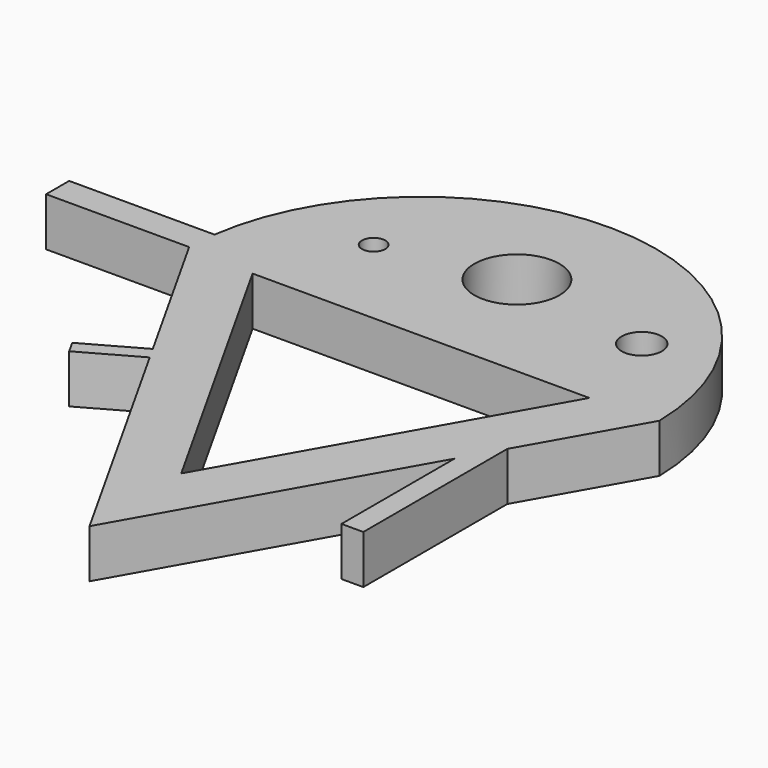
from build123d import *

# Parameters (mm, degrees)
F0_R     = 1.5262492047
F0_R_2   = 5.564877875
F0_R_3   = 2.6305534458
F1_DEPTH = 6.35


# Not quite as in the source:
# - a feature names something its author has since deleted; it is built from what else it names


with BuildPart() as f1:
    # F0 (on Top) → F1 (new body)
    with BuildSketch(Plane.XY):
        with BuildLine():
            Line((-18.5164521814, -21.5775697793), (0, -54.5748323202))
            Line((0, -54.5748323202), (19.7828651091, -19.6195188363))
            Line((19.7828651091, -19.6195188363), (22.6427465677, -14.5662541873))
            Line((22.6427465677, -14.5662541873), (30.8864787221, 0))
            ThreePointArc((30.8864787221, 0), (2.0232479541, 30.1763499671), (-30.3273923907, 3.7730498517))
            ThreePointArc((-30.3273923907, 3.7730498517), (-30.5341463656, 1.8911023526), (-30.6247305125, 0))
            Line((-30.6247305125, 0), (-19.4482157174, -19.9171196174))
            Line((-19.4482157174, -19.9171196174), (-18.5164521814, -21.5775697793))
        make_face()
        Polygon((22.1472843044, -0.5254783843), (0.0272358089, -39.6104756875), (-21.9053558016, -0.5254783843), (0.1308741048, -0.5254783843), align=None, mode=Mode.SUBTRACT)
        with Locations((-16.2284877151, 12.1713718399)):
            Circle(F0_R, mode=Mode.SUBTRACT)
        with Locations((0, 15.3123699129)):
            Circle(F0_R_2, mode=Mode.SUBTRACT)
        with Locations((18.8459847122, 12.1713718399)):
            Circle(F0_R_3, mode=Mode.SUBTRACT)
        Polygon((22.6427465677, -14.5662541873), (19.7828651091, -19.6195188363), (19.7828651091, -38.1040237844), (22.6427465677, -38.1040237844), align=None)
        Polygon((-25.7906284703, -25.6594822484), (-18.5164521814, -21.5775697793), (-19.4482157174, -19.9171196174), (-26.7223920062, -23.9990320865), align=None)
        with BuildLine():
            Line((-49.3409076612, 0), (-30.6247305125, 0))
            ThreePointArc((-30.6247305125, 0), (-30.5341463656, 1.8911023526), (-30.3273923907, 3.7730498517))
            Line((-30.3273923907, 3.7730498517), (-49.3409076612, 3.7730498517))
            Line((-49.3409076612, 3.7730498517), (-49.3409076612, 0))
        make_face()
    extrude(amount=F1_DEPTH)


solid = f1.part
